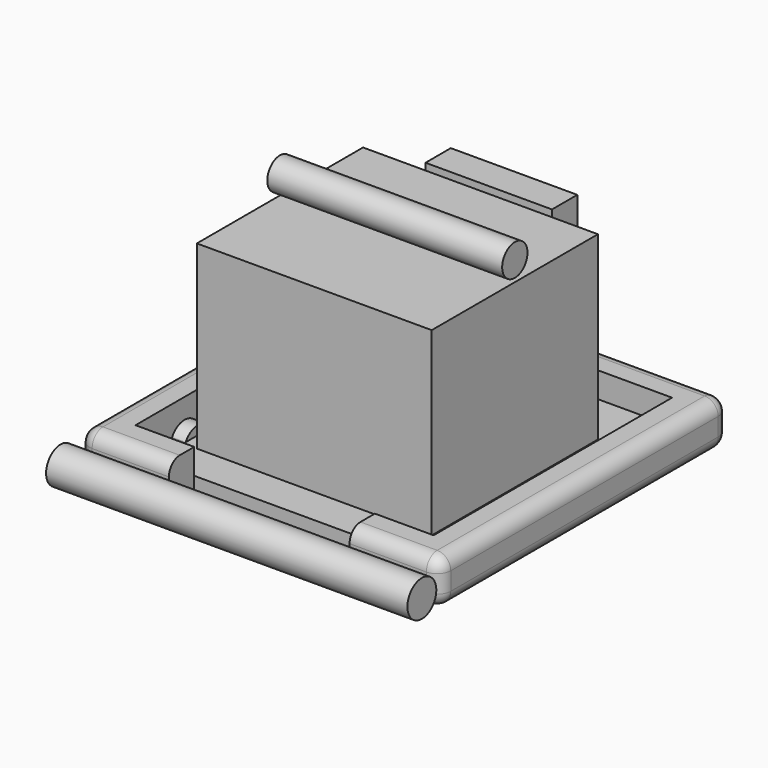
from build123d import *

# Parameters (mm, degrees)
F1_DEPTH      = 50.8
F3_DEPTH      = 38.1
F5_DEPTH      = 38.1
F11_T1_DEPTH  = 50.8
F11_S5_W      = 38.1
F11_S5_H      = 38.1
F11_T6_DEPTH  = 38.1
F11_S11_W     = 38.1
F11_S11_H     = 38.1
F11_T12_DEPTH = 38.1
F11_S17_W     = 38.1
F11_S17_H     = 38.1
F11_T18_DEPTH = 38.1
F11_S23_W     = 38.1
F11_S23_H     = 38.1
F11_T24_DEPTH = 38.1
F11_S29_W     = 38.1
F11_S29_H     = 38.1
F11_T30_DEPTH = 38.1
F11_S35_W     = 38.1
F11_S35_H     = 38.1
F11_T36_DEPTH = 38.1
F11_S41_W     = 38.1
F11_S41_H     = 38.1
F11_T42_DEPTH = 38.1
F11_S47_W     = 38.1
F11_S47_H     = 38.1
F11_T48_DEPTH = 38.1
F12_W         = 660.4
F12_H         = 584.2
F13_DEPTH     = 508
F14_R         = 76.2
F15_DEPTH     = 381
F16_W         = 355.6
F16_H         = 88.9
F17_DEPTH     = 508
F19_R         = 50.8
F20_DEPTH     = 1016
F21_R         = 44.45
F22_DEPTH     = 660.4


# Not quite as in the source:
# - a fillet or chamfer that OpenCascade refuses, or shapes differently, is made with other operations: its cross-section is extruded or revolved along the edge and cut away or added


with BuildPart() as f1:
    # F0 (on Top) → F1 (new body)
    with BuildSketch(Plane.XY):
        Polygon((371.4952406228, 636.845473688), (-466.7047593772, 636.845473688), (-466.7047593772, 586.045473688), (-415.9047593772, 586.045473688), (-415.9047593772, 374.3788070213), (-466.7047593772, 374.3788070213), (-466.7047593772, 323.5788070213), (-415.9047593772, 323.5788070213), (-415.9047593772, 111.9121403546), (-466.7047593772, 111.9121403546), (-466.7047593772, 61.1121403546), (-415.9047593772, 61.1121403546), (-415.9047593772, -150.554526312), (-466.7047593772, -150.554526312), (-466.7047593772, -201.354526312), (371.4952406228, -201.354526312), (371.4952406228, -150.554526312), (320.6952406228, -150.554526312), (320.6952406228, 61.1121403546), (371.4952406228, 61.1121403546), (371.4952406228, 111.9121403546), (320.6952406228, 111.9121403546), (320.6952406228, 323.5788070213), (371.4952406228, 323.5788070213), (371.4952406228, 374.3788070213), (320.6952406228, 374.3788070213), (320.6952406228, 586.045473688), (371.4952406228, 586.045473688), align=None)
    extrude(amount=F1_DEPTH)

    # F2 (on face) → F3 (join)
    with BuildSketch(Plane(origin=(-415.9047593772, 0, 0), x_dir=(0, -1, 0), z_dir=(-1, 0, 0))):
        with BuildLine():
            ThreePointArc((-173.7513831757, 50.8), (-217.745473688, 76.2), (-261.7395642002, 50.8))
            Line((-261.7395642002, 50.8), (-173.7513831757, 50.8))
        make_face()
        with BuildLine():
            ThreePointArc((-261.7395642002, 50.8), (-268.545473688, 25.4), (-261.7395642002, 0))
            Line((-261.7395642002, 0), (-173.7513831757, 0))
            ThreePointArc((-173.7513831757, 0), (-168.6764417125, 12.2519925088), (-166.945473688, 25.4))
            ThreePointArc((-166.945473688, 25.4), (-168.6764417125, 38.5480074912), (-173.7513831757, 50.8))
            Line((-173.7513831757, 50.8), (-261.7395642002, 50.8))
        make_face()
        with BuildLine():
            Line((-173.7513831757, 0), (-261.7395642002, 0))
            ThreePointArc((-261.7395642002, 0), (-217.745473688, -25.4), (-173.7513831757, 0))
        make_face()
        with BuildLine():
            ThreePointArc((88.715283491, 50.8), (44.7211929787, 76.2), (0.7271024665, 50.8))
            Line((0.7271024665, 50.8), (88.715283491, 50.8))
        make_face()
        with BuildLine():
            ThreePointArc((0.7271024665, 50.8), (-6.0788070213, 25.4), (0.7271024665, 0))
            Line((0.7271024665, 0), (88.715283491, 0))
            ThreePointArc((88.715283491, 0), (93.7902249542, 12.2519925088), (95.5211929787, 25.4))
            ThreePointArc((95.5211929787, 25.4), (93.7902249542, 38.5480074912), (88.715283491, 50.8))
            Line((88.715283491, 50.8), (0.7271024665, 50.8))
        make_face()
        with BuildLine():
            Line((88.715283491, 0), (0.7271024665, 0))
            ThreePointArc((0.7271024665, 0), (44.7211929787, -25.4), (88.715283491, 0))
        make_face()
        with BuildLine():
            ThreePointArc((-436.2180498424, 50.8), (-480.2121403546, 76.2), (-524.2062308669, 50.8))
            Line((-524.2062308669, 50.8), (-436.2180498424, 50.8))
        make_face()
        with BuildLine():
            Line((-436.2180498424, 0), (-524.2062308669, 0))
            ThreePointArc((-524.2062308669, 0), (-480.2121403546, -25.4), (-436.2180498424, 0))
        make_face()
        with BuildLine():
            ThreePointArc((-524.2062308669, 50.8), (-531.0121403546, 25.4), (-524.2062308669, 0))
            Line((-524.2062308669, 0), (-436.2180498424, 0))
            ThreePointArc((-436.2180498424, 0), (-431.1431083791, 12.2519925088), (-429.4121403546, 25.4))
            ThreePointArc((-429.4121403546, 25.4), (-431.1431083791, 38.5480074912), (-436.2180498424, 50.8))
            Line((-436.2180498424, 50.8), (-524.2062308669, 50.8))
        make_face()
    extrude(amount=F3_DEPTH)

    # F4 (on face) → F5 (join)
    with BuildSketch(Plane.YZ.offset(320.6952406228)):
        with BuildLine():
            ThreePointArc((-0.7271024665, 50.8), (-44.7211929787, 76.2), (-88.715283491, 50.8))
            Line((-88.715283491, 50.8), (-0.7271024665, 50.8))
        make_face()
        with BuildLine():
            ThreePointArc((-88.715283491, 50.8), (-95.5211929787, 25.4), (-88.715283491, 0))
            Line((-88.715283491, 0), (-0.7271024665, 0))
            ThreePointArc((-0.7271024665, 0), (4.3478389968, 12.2519925088), (6.0788070213, 25.4))
            ThreePointArc((6.0788070213, 25.4), (4.3478389968, 38.5480074912), (-0.7271024665, 50.8))
            Line((-0.7271024665, 50.8), (-88.715283491, 50.8))
        make_face()
        with BuildLine():
            Line((-0.7271024665, 0), (-88.715283491, 0))
            ThreePointArc((-88.715283491, 0), (-44.7211929787, -25.4), (-0.7271024665, 0))
        make_face()
        with BuildLine():
            ThreePointArc((261.7395642002, 50.8), (217.745473688, 76.2), (173.7513831757, 50.8))
            Line((173.7513831757, 50.8), (261.7395642002, 50.8))
        make_face()
        with BuildLine():
            ThreePointArc((173.7513831757, 50.8), (166.945473688, 25.4), (173.7513831757, 0))
            Line((173.7513831757, 0), (261.7395642002, 0))
            ThreePointArc((261.7395642002, 0), (266.8145056634, 12.2519925088), (268.545473688, 25.4))
            ThreePointArc((268.545473688, 25.4), (266.8145056634, 38.5480074912), (261.7395642002, 50.8))
            Line((261.7395642002, 50.8), (173.7513831757, 50.8))
        make_face()
        with BuildLine():
            Line((261.7395642002, 0), (173.7513831757, 0))
            ThreePointArc((173.7513831757, 0), (217.745473688, -25.4), (261.7395642002, 0))
        make_face()
        with BuildLine():
            ThreePointArc((524.2062308669, 50.8), (480.2121403546, 76.2), (436.2180498424, 50.8))
            Line((436.2180498424, 50.8), (524.2062308669, 50.8))
        make_face()
        with BuildLine():
            ThreePointArc((436.2180498424, 50.8), (429.4121403546, 25.4), (436.2180498424, 0))
            Line((436.2180498424, 0), (524.2062308669, 0))
            ThreePointArc((524.2062308669, 0), (529.2811723301, 12.2519925088), (531.0121403546, 25.4))
            ThreePointArc((531.0121403546, 25.4), (529.2811723301, 38.5480074912), (524.2062308669, 50.8))
            Line((524.2062308669, 50.8), (436.2180498424, 50.8))
        make_face()
        with BuildLine():
            Line((524.2062308669, 0), (436.2180498424, 0))
            ThreePointArc((436.2180498424, 0), (480.2121403546, -25.4), (524.2062308669, 0))
        make_face()
    extrude(amount=F5_DEPTH)


with BuildPart() as f10:
    # F10: sweep along a path in F7
    with BuildLine(Plane.XY.offset(50.8)) as f10_path:
        Line((206.3952406228, -245.804526312), (415.9452406228, -245.804526312))
        Line((415.9452406228, -245.804526312), (415.9452406228, 681.295473688))
        Line((415.9452406228, 681.295473688), (-511.1547593772, 681.295473688))
        Line((-511.1547593772, 681.295473688), (-511.1547593772, -245.804526312))
        Line((-511.1547593772, -245.804526312), (-301.6047593772, -245.804526312))
    # F9 (on line) → F10 (sweep)
    with BuildSketch(Plane.YZ.offset(206.3952406228)):
        with BuildLine():
            Line((-201.354526312, 0), (-201.354526312, 50.8))
            Line((-201.354526312, 50.8), (-201.354526312, 122.3268861175))
            Line((-201.354526312, 122.3268861175), (-252.154526312, 122.3268861175))
            ThreePointArc((-252.154526312, 122.3268861175), (-279.0952946752, 111.1676544807), (-290.254526312, 84.2268861175))
            Line((-290.254526312, 84.2268861175), (-290.254526312, 33.4268861175))
            ThreePointArc((-290.254526312, 33.4268861175), (-279.0952946752, 6.4861177543), (-252.154526312, -4.6731138825))
            Line((-252.154526312, -4.6731138825), (-201.354526312, -4.6731138825))
            Line((-201.354526312, -4.6731138825), (-201.354526312, 0))
        make_face()
    sweep(path=f10_path.line, transition=Transition.RIGHT)

    # F11: fillet of radius 38.1 on 4 edges, made by hand

    # F11_s2 → F11_t1 (cut)
    with BuildSketch(Plane.XY.offset(33.4268861175)):
        with BuildLine():
            ThreePointArc((-555.6047593772, -252.154526312), (-544.4455277404, -279.0952946752), (-517.5047593772, -290.254526312))
            Line((-517.5047593772, -290.254526312), (-555.6047593772, -290.254526312))
            Line((-555.6047593772, -290.254526312), (-555.6047593772, -252.154526312))
        make_face()
        with BuildLine():
            ThreePointArc((460.3952406228, -252.154526312), (449.236008986, -279.0952946752), (422.2952406228, -290.254526312))
            Line((422.2952406228, -290.254526312), (460.3952406228, -290.254526312))
            Line((460.3952406228, -290.254526312), (460.3952406228, -252.154526312))
        make_face()
        with BuildLine():
            ThreePointArc((460.3952406228, 687.645473688), (449.236008986, 714.5862420512), (422.2952406228, 725.745473688))
            Line((422.2952406228, 725.745473688), (460.3952406228, 725.745473688))
            Line((460.3952406228, 725.745473688), (460.3952406228, 687.645473688))
        make_face()
        with BuildLine():
            ThreePointArc((-517.5047593772, 725.745473688), (-544.4455277404, 714.5862420512), (-555.6047593772, 687.645473688))
            Line((-555.6047593772, 687.645473688), (-555.6047593772, 725.745473688))
            Line((-555.6047593772, 725.745473688), (-517.5047593772, 725.745473688))
        make_face()
    extrude(amount=F11_T1_DEPTH, mode=Mode.SUBTRACT)


with BuildPart() as f11_tool4:
    # F11_s5 → F11_t6 (new body)
    with BuildSketch(Plane.XZ.offset(-687.645473688)):
        with Locations((-536.5547593772, 14.3768861175)):
            Rectangle(F11_S5_W, F11_S5_H)
    extrude(amount=-F11_T6_DEPTH)

    # F11_s7 → F11_t8 (revolve, cut)
    with BuildSketch(Plane(origin=(-517.5047593772, 687.645473688, 33.4268861175), x_dir=(0.7071067812, 0, 0.7071067812), z_dir=(-0.7071067812, 0, 0.7071067812))):
        with BuildLine():
            ThreePointArc((0, -38.1), (38.1, 0), (0, 38.1))
            Line((0, 38.1), (0, -38.1))
        make_face()
    revolve(axis=Axis((-517.5047593772, 687.645473688, 33.4268861175), (0, 1, 0)), mode=Mode.SUBTRACT)


with BuildPart() as f10_1:
    add(f10.part)

    # F11_t3: cut F11_tool4
    add(f11_tool4.part, mode=Mode.SUBTRACT)


with BuildPart() as f11_tool10:
    # F11_s11 → F11_t12 (new body)
    with BuildSketch(Plane.XZ.offset(-687.645473688)):
        with Locations((-536.5547593772, 103.2768861175)):
            Rectangle(F11_S11_W, F11_S11_H)
    extrude(amount=-F11_T12_DEPTH)

    # F11_s13 → F11_t14 (revolve, cut)
    with BuildSketch(Plane(origin=(-517.5047593772, 687.645473688, 84.2268861175), x_dir=(0.7071067812, 0, -0.7071067812), z_dir=(0.7071067812, 0, 0.7071067812))):
        with BuildLine():
            ThreePointArc((0, -38.1), (38.1, 0), (0, 38.1))
            Line((0, 38.1), (0, -38.1))
        make_face()
    revolve(axis=Axis((-517.5047593772, 687.645473688, 84.2268861175), (0, 1, 0)), mode=Mode.SUBTRACT)


with BuildPart() as f10_2:
    add(f10_1.part)

    # F11_t9: cut F11_tool10
    add(f11_tool10.part, mode=Mode.SUBTRACT)


with BuildPart() as f11_tool16:
    # F11_s17 → F11_t18 (new body)
    with BuildSketch(Plane.YZ.offset(422.2952406228)):
        with Locations((706.695473688, 14.3768861175)):
            Rectangle(F11_S17_W, F11_S17_H)
    extrude(amount=F11_T18_DEPTH)

    # F11_s19 → F11_t20 (revolve, cut)
    with BuildSketch(Plane(origin=(422.2952406228, 687.645473688, 33.4268861175), x_dir=(0, -0.7071067812, 0.7071067812), z_dir=(0, 0.7071067812, 0.7071067812))):
        with BuildLine():
            ThreePointArc((0, -38.1), (38.1, 0), (0, 38.1))
            Line((0, 38.1), (0, -38.1))
        make_face()
    revolve(axis=Axis((422.2952406228, 687.645473688, 33.4268861175), (1, 0, 0)), mode=Mode.SUBTRACT)


with BuildPart() as f10_3:
    add(f10_2.part)

    # F11_t15: cut F11_tool16
    add(f11_tool16.part, mode=Mode.SUBTRACT)


with BuildPart() as f11_tool22:
    # F11_s23 → F11_t24 (new body)
    with BuildSketch(Plane.YZ.offset(422.2952406228)):
        with Locations((706.695473688, 103.2768861175)):
            Rectangle(F11_S23_W, F11_S23_H)
    extrude(amount=F11_T24_DEPTH)

    # F11_s25 → F11_t26 (revolve, cut)
    with BuildSketch(Plane(origin=(422.2952406228, 687.645473688, 84.2268861175), x_dir=(0, -0.7071067812, -0.7071067812), z_dir=(0, -0.7071067812, 0.7071067812))):
        with BuildLine():
            ThreePointArc((0, -38.1), (38.1, 0), (0, 38.1))
            Line((0, 38.1), (0, -38.1))
        make_face()
    revolve(axis=Axis((422.2952406228, 687.645473688, 84.2268861175), (1, 0, 0)), mode=Mode.SUBTRACT)


with BuildPart() as f10_4:
    add(f10_3.part)

    # F11_t21: cut F11_tool22
    add(f11_tool22.part, mode=Mode.SUBTRACT)


with BuildPart() as f11_tool28:
    # F11_s29 → F11_t30 (new body)
    with BuildSketch(Plane.YZ.offset(422.2952406228)):
        with Locations((-271.204526312, 14.3768861175)):
            Rectangle(F11_S29_W, F11_S29_H)
    extrude(amount=F11_T30_DEPTH)

    # F11_s31 → F11_t32 (revolve, cut)
    with BuildSketch(Plane(origin=(422.2952406228, -252.154526312, 33.4268861175), x_dir=(0, 0.7071067812, 0.7071067812), z_dir=(0, 0.7071067812, -0.7071067812))):
        with BuildLine():
            ThreePointArc((0, -38.1), (38.1, 0), (0, 38.1))
            Line((0, 38.1), (0, -38.1))
        make_face()
    revolve(axis=Axis((422.2952406228, -252.154526312, 33.4268861175), (1, 0, 0)), mode=Mode.SUBTRACT)


with BuildPart() as f10_5:
    add(f10_4.part)

    # F11_t27: cut F11_tool28
    add(f11_tool28.part, mode=Mode.SUBTRACT)


with BuildPart() as f11_tool34:
    # F11_s35 → F11_t36 (new body)
    with BuildSketch(Plane.YZ.offset(422.2952406228)):
        with Locations((-271.204526312, 103.2768861175)):
            Rectangle(F11_S35_W, F11_S35_H)
    extrude(amount=F11_T36_DEPTH)

    # F11_s37 → F11_t38 (revolve, cut)
    with BuildSketch(Plane(origin=(422.2952406228, -252.154526312, 84.2268861175), x_dir=(0, 0.7071067812, -0.7071067812), z_dir=(0, -0.7071067812, -0.7071067812))):
        with BuildLine():
            ThreePointArc((0, -38.1), (38.1, 0), (0, 38.1))
            Line((0, 38.1), (0, -38.1))
        make_face()
    revolve(axis=Axis((422.2952406228, -252.154526312, 84.2268861175), (1, 0, 0)), mode=Mode.SUBTRACT)


with BuildPart() as f10_6:
    add(f10_5.part)

    # F11_t33: cut F11_tool34
    add(f11_tool34.part, mode=Mode.SUBTRACT)


with BuildPart() as f11_tool40:
    # F11_s41 → F11_t42 (new body)
    with BuildSketch(Plane.YZ.offset(-517.5047593772)):
        with Locations((-271.204526312, 14.3768861175)):
            Rectangle(F11_S41_W, F11_S41_H)
    extrude(amount=-F11_T42_DEPTH)

    # F11_s43 → F11_t44 (revolve, cut)
    with BuildSketch(Plane(origin=(-517.5047593772, -252.154526312, 33.4268861175), x_dir=(0, 0.7071067812, 0.7071067812), z_dir=(0, -0.7071067812, 0.7071067812))):
        with BuildLine():
            ThreePointArc((0, -38.1), (38.1, 0), (0, 38.1))
            Line((0, 38.1), (0, -38.1))
        make_face()
    revolve(axis=Axis((-517.5047593772, -252.154526312, 33.4268861175), (-1, 0, 0)), mode=Mode.SUBTRACT)


with BuildPart() as f10_7:
    add(f10_6.part)

    # F11_t39: cut F11_tool40
    add(f11_tool40.part, mode=Mode.SUBTRACT)


with BuildPart() as f11_tool46:
    # F11_s47 → F11_t48 (new body)
    with BuildSketch(Plane.YZ.offset(-517.5047593772)):
        with Locations((-271.204526312, 103.2768861175)):
            Rectangle(F11_S47_W, F11_S47_H)
    extrude(amount=-F11_T48_DEPTH)

    # F11_s49 → F11_t50 (revolve, cut)
    with BuildSketch(Plane(origin=(-517.5047593772, -252.154526312, 84.2268861175), x_dir=(0, 0.7071067812, -0.7071067812), z_dir=(0, 0.7071067812, 0.7071067812))):
        with BuildLine():
            ThreePointArc((0, -38.1), (38.1, 0), (0, 38.1))
            Line((0, 38.1), (0, -38.1))
        make_face()
    revolve(axis=Axis((-517.5047593772, -252.154526312, 84.2268861175), (-1, 0, 0)), mode=Mode.SUBTRACT)


with BuildPart() as f10_8:
    add(f10_7.part)

    # F11_t45: cut F11_tool46
    add(f11_tool46.part, mode=Mode.SUBTRACT)


with BuildPart() as f13:
    # F12 (on face) → F13 (new body)
    with BuildSketch(Plane.XY.offset(50.8)):
        with Locations((-47.6047593772, 195.2356742796)):
            Rectangle(F12_W, F12_H)
    extrude(amount=F13_DEPTH)


with BuildPart() as f15:
    # F14 (on face) → F15 (new body)
    with BuildSketch(Plane.XY.offset(50.8)):
        with Locations((-47.6047593772, 30.1356742796)):
            Circle(F14_R)
    extrude(amount=F15_DEPTH)


with BuildPart() as f17:
    # F16 (on face) → F17 (new body)
    with BuildSketch(Plane.XY.offset(50.8)):
        with Locations((-47.6047593772, 560.8344823837)):
            Rectangle(F16_W, F16_H)
    extrude(amount=F17_DEPTH)


with BuildPart() as f20:
    # F19 (on offset) → F20 (new body, through all)
    with BuildSketch(Plane(origin=(-555.6047593772, 0, 0), x_dir=(0, -1, 0), z_dir=(-1, 0, 0))):
        with Locations((353.7409305573, 57.0096969604)):
            Circle(F19_R)
    extrude(amount=-F20_DEPTH)


with BuildPart() as f22:
    # F21 (on face) → F22 (new body, through all)
    with BuildSketch(Plane(origin=(-377.8047593772, 0, 0), x_dir=(0, -1, 0), z_dir=(-1, 0, 0))):
        with Locations((-195.2356742796, 613.7475967407)):
            Circle(F21_R)
    extrude(amount=-F22_DEPTH)


solid = Compound([f1.part, f10_8.part, f13.part, f15.part, f17.part, f20.part, f22.part])
